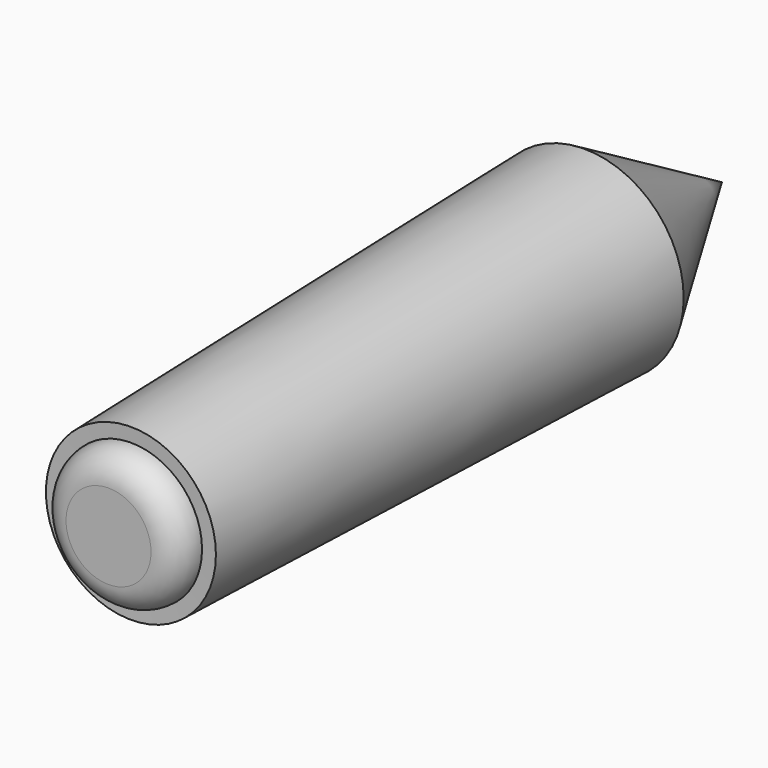
from build123d import *

# Parameters (mm, degrees)
F2_R = 3.99999


# Not quite as in the source:
# - a fillet or chamfer is up to 0.001 mm smaller than in the source, because OpenCascade refuses the exact size


with BuildPart() as f1:
    # F0 (on Top) → F1 (revolve)
    with BuildSketch(Plane.XY):
        Polygon((14, 29.3282374667), (0, 53.5769487726), (0, -54.6717625333), (10, -54.6717625333), (10, -50.6717625333), (12, -50.7217313223), align=None)
    revolve(axis=Axis((0, -0.5474068804, 0), (0, 1, 0)))

    # F2 (radius 4 in the source; OpenCascade refuses exactly that, so slightly less here)
    f2_edges = [f1.edges().sort_by_distance(p)[0] for p in [
        (-10, -54.671763, 0),
    ]]
    fillet(f2_edges, radius=F2_R)


solid = f1.part
